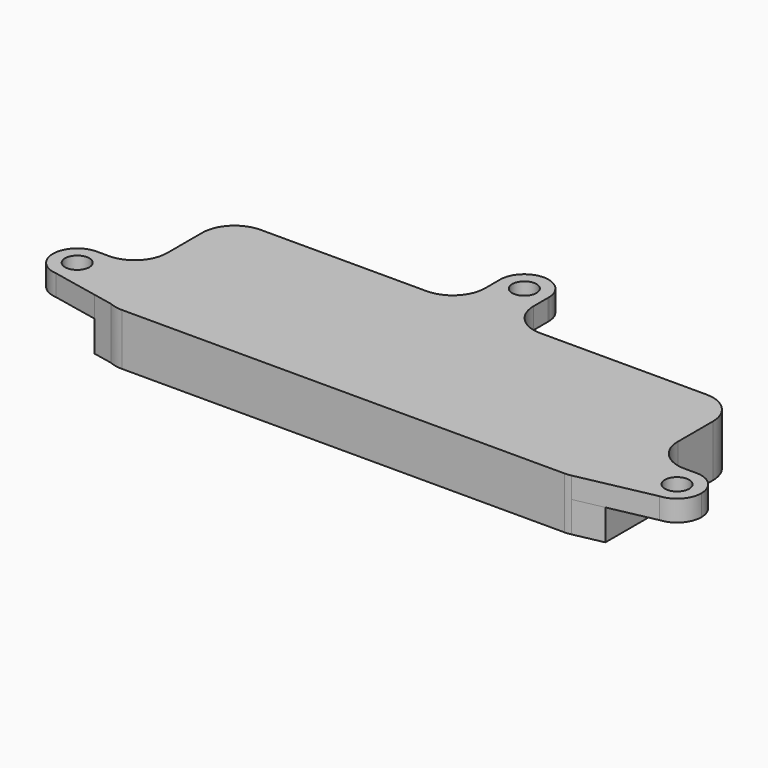
from build123d import *

# Parameters (mm, degrees)
F0_R     = 1.905
F1_DEPTH = 3.302
F3_DEPTH = 4.826
F5_DEPTH = 4.826


# Not quite as in the source:
# - a feature names something its author has since deleted; it is built from what else it names


with BuildPart() as f1:
    # F0 (on Top) → F1 (new body)
    with BuildSketch(Plane.XY):
        with BuildLine():
            Line((-8.8801402367, 13.589), (-34.925, 13.589))
            ThreePointArc((-34.925, 13.589), (-38.5171024484, 12.1011024484), (-40.005, 8.509))
            Line((-40.005, 8.509), (-40.005, 1.6507252969))
            Line((-40.005, 1.6507252969), (-40.005, -12.5406651425))
            Line((-40.005, -12.5406651425), (-36.9360269804, -13.1739941569))
            ThreePointArc((-36.9360269804, -13.1739941569), (-35.9517009503, -13.4841668473), (-34.925, -13.589))
            Line((-34.925, -13.589), (34.4062974357, -13.589))
            ThreePointArc((34.4062974357, -13.589), (34.9223170166, -13.562723755), (35.4329983861, -13.4841668473))
            Line((35.4329983861, -13.4841668473), (47.2909788792, -11.0370931682))
            ThreePointArc((47.2909788792, -11.0370931682), (43.1839507681, -7.4124625154), (46.9442489114, -3.4292747031))
            Line((46.9442489114, -3.4292747031), (45.085, -3.4292747031))
            ThreePointArc((45.085, -3.4292747031), (41.4928975516, -1.9413771515), (40.005, 1.6507252969))
            Line((40.005, 1.6507252969), (40.005, 8.509))
            ThreePointArc((40.005, 8.509), (38.5171024484, 12.1011024484), (34.925, 13.589))
            Line((34.925, 13.589), (8.8801402367, 13.589))
            ThreePointArc((8.8801402367, 13.589), (5.2880377883, 15.0768975516), (3.8001402367, 18.669))
            Line((3.8001402367, 18.669), (3.8001402367, 21.4595748034))
            ThreePointArc((3.8001402367, 21.4595748034), (0, 17.7876222504), (-3.8001402367, 21.4595748034))
            Line((-3.8001402367, 21.4595748034), (-3.8001402367, 18.669))
            ThreePointArc((-3.8001402367, 18.669), (-5.2880377883, 15.0768975516), (-8.8801402367, 13.589))
        make_face()
        with BuildLine():
            Line((-40.005, -12.5406651425), (-40.005, 1.6507252969))
            ThreePointArc((-40.005, 1.6507252969), (-41.4928975516, -1.9413771515), (-45.085, -3.4292747031))
            Line((-45.085, -3.4292747031), (-46.9442489114, -3.4292747031))
            ThreePointArc((-46.9442489114, -3.4292747031), (-44.2797959812, -4.5611474693), (-43.18, -7.239))
            ThreePointArc((-43.18, -7.239), (-44.4045241763, -10.0374665024), (-47.2909788792, -11.0370931682))
            Line((-47.2909788792, -11.0370931682), (-40.005, -12.5406651425))
        make_face()
        with BuildLine():
            Line((-3.8001402367, 21.7204251966), (-3.8001402367, 21.4595748034))
            ThreePointArc((-3.8001402367, 21.4595748034), (0, 17.7876222504), (3.8001402367, 21.4595748034))
            Line((3.8001402367, 21.4595748034), (3.8001402367, 21.7204251966))
            ThreePointArc((3.8001402367, 21.7204251966), (0, 25.3923777496), (-3.8001402367, 21.7204251966))
        make_face()
        with Locations((0, 21.59)):
            Circle(F0_R, mode=Mode.SUBTRACT)
        with BuildLine():
            ThreePointArc((-3.8001402367, 21.7204251966), (-3.8023777496, 21.59), (-3.8001402367, 21.4595748034))
            Line((-3.8001402367, 21.4595748034), (-3.8001402367, 21.7204251966))
        make_face()
        with BuildLine():
            Line((3.8001402367, 21.7204251966), (3.8001402367, 21.4595748034))
            ThreePointArc((3.8001402367, 21.4595748034), (3.8018183303, 21.524777806), (3.8023777496, 21.59))
            ThreePointArc((3.8023777496, 21.59), (3.8018183303, 21.655222194), (3.8001402367, 21.7204251966))
        make_face()
        with BuildLine():
            Line((-47.0357510886, -3.4292747031), (-46.9442489114, -3.4292747031))
            ThreePointArc((-46.9442489114, -3.4292747031), (-46.99, -3.429), (-47.0357510886, -3.4292747031))
        make_face()
        with BuildLine():
            ThreePointArc((-43.18, -7.239), (-44.2797959812, -4.5611474693), (-46.9442489114, -3.4292747031))
            Line((-46.9442489114, -3.4292747031), (-47.0357510886, -3.4292747031))
            ThreePointArc((-47.0357510886, -3.4292747031), (-50.7978577793, -7.1112536385), (-47.2909788792, -11.0370931682))
            ThreePointArc((-47.2909788792, -11.0370931682), (-44.4045241763, -10.0374665024), (-43.18, -7.239))
        make_face()
        with Locations((-46.99, -7.239)):
            Circle(F0_R, mode=Mode.SUBTRACT)
        with BuildLine():
            ThreePointArc((46.9442489114, -3.4292747031), (43.1839507681, -7.4124625154), (47.2909788792, -11.0370931682))
            ThreePointArc((47.2909788792, -11.0370931682), (49.7884665024, -9.8244758237), (50.8, -7.239))
            ThreePointArc((50.8, -7.239), (49.7002040188, -4.5611474693), (47.0357510886, -3.4292747031))
            Line((47.0357510886, -3.4292747031), (46.9442489114, -3.4292747031))
        make_face()
        with Locations((46.99, -7.239)):
            Circle(F0_R, mode=Mode.SUBTRACT)
        with BuildLine():
            ThreePointArc((47.0357510886, -3.4292747031), (46.99, -3.429), (46.9442489114, -3.4292747031))
            Line((46.9442489114, -3.4292747031), (47.0357510886, -3.4292747031))
        make_face()
    extrude(amount=F1_DEPTH)

    # F2 (on face) → F3 (join)
    with BuildSketch(Plane(origin=(0, 0, 0), x_dir=(1, 0, 0), z_dir=(0, 0, -1))):
        with BuildLine():
            Line((-40.005, -1.6507252969), (-40.005, -5.0798626485))
            Line((-40.005, -5.0798626485), (-40.005, -8.509))
            ThreePointArc((-40.005, -8.509), (-38.5171024484, -12.1011024484), (-34.925, -13.589))
            Line((-34.925, -13.589), (-13.1316846237, -13.589))
            Line((-13.1316846237, -13.589), (-8.8801402367, -13.589))
            Line((-8.8801402367, -13.589), (8.8801402367, -13.589))
            Line((8.8801402367, -13.589), (9.6433609724, -13.589))
            Line((9.6433609724, -13.589), (34.925, -13.589))
            ThreePointArc((34.925, -13.589), (38.5171024484, -12.1011024484), (40.005, -8.509))
            Line((40.005, -8.509), (40.005, -5.0798626485))
            Line((40.005, -5.0798626485), (40.005, -1.6507252969))
            Line((40.005, -1.6507252969), (40.005, 12.5406651425))
            Line((40.005, 12.5406651425), (35.4329983861, 13.4841668473))
            ThreePointArc((35.4329983861, 13.4841668473), (34.9223170166, 13.562723755), (34.4062974357, 13.589))
            Line((34.4062974357, 13.589), (-34.925, 13.589))
            ThreePointArc((-34.925, 13.589), (-35.9517009503, 13.4841668473), (-36.9360269804, 13.1739941569))
            Line((-36.9360269804, 13.1739941569), (-40.005, 12.5406651425))
            Line((-40.005, 12.5406651425), (-40.005, -1.6507252969))
        make_face()
    extrude(amount=F3_DEPTH)

    # F4 (on face) → F5 (cut)
    with BuildSketch(Plane(origin=(0, 0, -4.826), x_dir=(1, 0, 0), z_dir=(0, 0, -1))):
        with BuildLine():
            ThreePointArc((-34.9554307759, 4.0977204838), (-34.583456388, 3.1996948717), (-33.6854307759, 2.8277204838))
            Line((-33.6854307759, 2.8277204838), (-3.7169939526, 2.8277204838))
            ThreePointArc((-3.7169939526, 2.8277204838), (-2.8189683405, 3.1996948717), (-2.4469939526, 4.0977204838))
            Line((-2.4469939526, 4.0977204838), (-2.4469939526, 9.3762063268))
            ThreePointArc((-2.4469939526, 9.3762063268), (-2.8189683405, 10.2742319389), (-3.7169939526, 10.6462063268))
            Line((-3.7169939526, 10.6462063268), (-33.6854307759, 10.6462063268))
            ThreePointArc((-33.6854307759, 10.6462063268), (-34.583456388, 10.2742319389), (-34.9554307759, 9.3762063268))
            Line((-34.9554307759, 9.3762063268), (-34.9554307759, 4.0977204838))
        make_face()
        with BuildLine():
            ThreePointArc((3.7169939526, 10.6462063268), (2.8189683405, 10.2742319389), (2.4469939526, 9.3762063268))
            Line((2.4469939526, 9.3762063268), (2.4469939526, 4.0977204838))
            ThreePointArc((2.4469939526, 4.0977204838), (2.8189683405, 3.1996948717), (3.7169939526, 2.8277204838))
            Line((3.7169939526, 2.8277204838), (33.6854307759, 2.8277204838))
            ThreePointArc((33.6854307759, 2.8277204838), (34.583456388, 3.1996948717), (34.9554307759, 4.0977204838))
            Line((34.9554307759, 4.0977204838), (34.9554307759, 9.3762063268))
            ThreePointArc((34.9554307759, 9.3762063268), (34.583456388, 10.2742319389), (33.6854307759, 10.6462063268))
            Line((33.6854307759, 10.6462063268), (3.7169939526, 10.6462063268))
        make_face()
        with BuildLine():
            Line((-3.7169939526, -2.8277204838), (-33.6854307759, -2.8277204838))
            ThreePointArc((-33.6854307759, -2.8277204838), (-34.583456388, -3.1996948717), (-34.9554307759, -4.0977204838))
            Line((-34.9554307759, -4.0977204838), (-34.9554307759, -9.3762063268))
            ThreePointArc((-34.9554307759, -9.3762063268), (-34.583456388, -10.2742319389), (-33.6854307759, -10.6462063268))
            Line((-33.6854307759, -10.6462063268), (-3.7169939526, -10.6462063268))
            ThreePointArc((-3.7169939526, -10.6462063268), (-2.8189683405, -10.2742319389), (-2.4469939526, -9.3762063268))
            Line((-2.4469939526, -9.3762063268), (-2.4469939526, -4.0977204838))
            ThreePointArc((-2.4469939526, -4.0977204838), (-2.8189683405, -3.1996948717), (-3.7169939526, -2.8277204838))
        make_face()
        with BuildLine():
            Line((2.4469939526, -4.0977204838), (2.4469939526, -9.3762063268))
            ThreePointArc((2.4469939526, -9.3762063268), (2.8189683405, -10.2742319389), (3.7169939526, -10.6462063268))
            Line((3.7169939526, -10.6462063268), (33.6854307759, -10.6462063268))
            ThreePointArc((33.6854307759, -10.6462063268), (34.583456388, -10.2742319389), (34.9554307759, -9.3762063268))
            Line((34.9554307759, -9.3762063268), (34.9554307759, -4.0977204838))
            ThreePointArc((34.9554307759, -4.0977204838), (34.583456388, -3.1996948717), (33.6854307759, -2.8277204838))
            Line((33.6854307759, -2.8277204838), (3.7169939526, -2.8277204838))
            ThreePointArc((3.7169939526, -2.8277204838), (2.8189683405, -3.1996948717), (2.4469939526, -4.0977204838))
        make_face()
    extrude(amount=-F5_DEPTH, mode=Mode.SUBTRACT)


solid = f1.part
